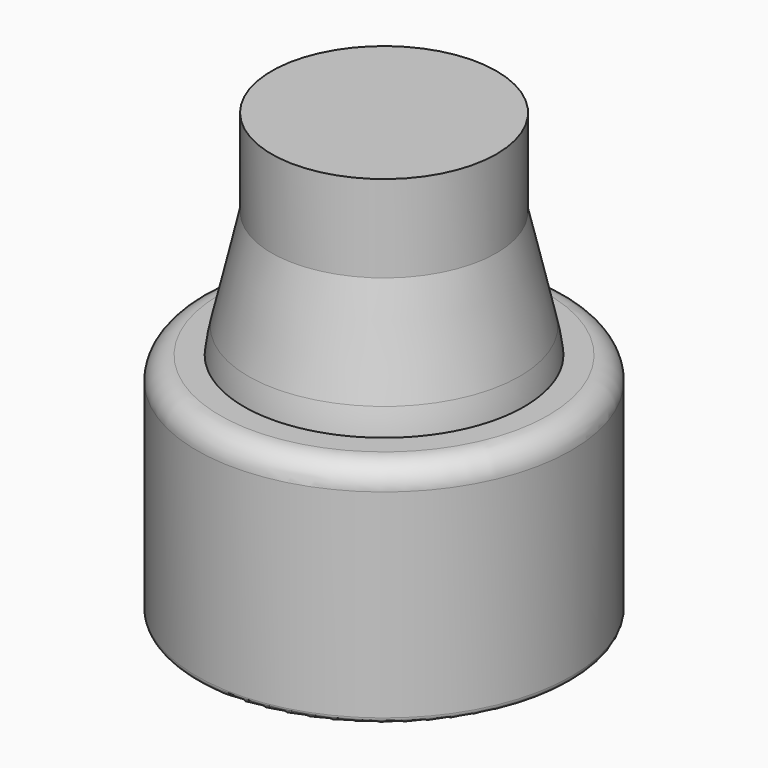
from build123d import *

# Parameters (mm, degrees)
F2_R     = 4.2825511293
F3_DEPTH = 7.85
F4_R     = 4
F5_DEPTH = 1
F5_TAPER = 70


# Not quite as in the source:
# - an extrude ends at something that could not be found from the text; its depth is read off the source's solid


with BuildPart() as f1:
    # F0 (on Front) → F1 (revolve)
    with BuildSketch(Plane.XZ):
        with BuildLine():
            Line((5.65, 7.85), (4, 7.85))
            Line((4, 7.85), (4, 4.75))
            Line((4, 4.75), (1.25, 3.1622867597))
            Line((1.25, 3.1622867597), (0, 3.1622867597))
            Line((0, 3.1622867597), (0, 0))
            Line((0, 0), (6.25, 0))
            ThreePointArc((6.25, 0), (6.3914213562, 0.0585786438), (6.45, 0.2))
            Line((6.45, 0.2), (6.45, 7.05))
            ThreePointArc((6.45, 7.05), (6.2156854249, 7.6156854249), (5.65, 7.85))
        make_face()
    revolve(axis=Axis((0, 0, 1.5811433799), (0, 0, -1)))

    # F2 (on face) → F3 (join, through all)
    with BuildSketch(Plane.XY.offset(7.85)):
        Circle(F2_R)
        with BuildLine():
            ThreePointArc((-0.772740661, 3.4070552361), (0, 4), (0.772740661, 3.4070552361))
            Line((0.772740661, 3.4070552361), (0.7889794079, 3.3464514079))
            ThreePointArc((0.7889794079, 3.3464514079), (1.4412755647, 2.4963625057), (2.5036222278, 2.3565019142))
            Line((2.5036222278, 2.3565019142), (2.564226056, 2.372740661))
            ThreePointArc((2.564226056, 2.372740661), (3.4641016151, 2), (3.3369667171, 1.0343145751))
            Line((3.3369667171, 1.0343145751), (3.2926016357, 0.9899494937))
            ThreePointArc((3.2926016357, 0.9899494937), (2.8825511293, 0), (3.2926016357, -0.9899494937))
            Line((3.2926016357, -0.9899494937), (3.3369667171, -1.0343145751))
            ThreePointArc((3.3369667171, -1.0343145751), (3.4641016151, -2), (2.564226056, -2.372740661))
            Line((2.564226056, -2.372740661), (2.5036222278, -2.3565019142))
            ThreePointArc((2.5036222278, -2.3565019142), (1.4412755647, -2.4963625057), (0.7889794079, -3.3464514079))
            Line((0.7889794079, -3.3464514079), (0.772740661, -3.4070552361))
            ThreePointArc((0.772740661, -3.4070552361), (0, -4), (-0.772740661, -3.4070552361))
            Line((-0.772740661, -3.4070552361), (-0.7889794079, -3.3464514079))
            ThreePointArc((-0.7889794079, -3.3464514079), (-1.4412755647, -2.4963625057), (-2.5036222278, -2.3565019142))
            Line((-2.5036222278, -2.3565019142), (-2.564226056, -2.372740661))
            ThreePointArc((-2.564226056, -2.372740661), (-3.4641016151, -2), (-3.3369667171, -1.0343145751))
            Line((-3.3369667171, -1.0343145751), (-3.2926016357, -0.9899494937))
            ThreePointArc((-3.2926016357, -0.9899494937), (-2.8825511293, 0), (-3.2926016357, 0.9899494937))
            Line((-3.2926016357, 0.9899494937), (-3.3369667171, 1.0343145751))
            ThreePointArc((-3.3369667171, 1.0343145751), (-3.4641016151, 2), (-2.564226056, 2.372740661))
            Line((-2.564226056, 2.372740661), (-2.5036222278, 2.3565019142))
            ThreePointArc((-2.5036222278, 2.3565019142), (-1.4412755647, 2.4963625057), (-0.7889794079, 3.3464514079))
            Line((-0.7889794079, 3.3464514079), (-0.772740661, 3.4070552361))
        make_face(mode=Mode.SUBTRACT)
    extrude(amount=-F3_DEPTH)

    # F4 (on face) → F5 (cut)
    with BuildSketch(Plane.XY.offset(7.85)):
        Circle(F4_R)
    extrude(amount=-F5_DEPTH, taper=F5_TAPER, mode=Mode.SUBTRACT)


with BuildPart() as f7:
    # F6 (on Front) → F7 (revolve)
    with BuildSketch(Plane.XZ):
        with BuildLine():
            Line((3.875, 15.2), (0, 15.2))
            Line((0, 15.2), (0, 0))
            Line((0, 0), (3.495, 0))
            Line((3.495, 0), (4.6778236218, 5.1233719814))
            ThreePointArc((4.6778236218, 5.1233719814), (4.8828631035, 6.9229804161), (4.6778236218, 8.7225888509))
            Line((4.6778236218, 8.7225888509), (3.875, 12.2))
            Line((3.875, 12.2), (3.875, 15.2))
        make_face()
    revolve(axis=Axis((0, 0, 7.6), (0, 0, -1)))


with BuildPart() as f9:
    # F8 (on Front) → F9 (revolve)
    with BuildSketch(Plane.XZ):
        with BuildLine():
            Line((0, 7.0269373127), (0, 0))
            Line((0, 0), (5.3425146232, 0))
            ThreePointArc((5.3425146232, 0), (5.679504679, 0.1306252549), (5.840417087, 0.4542491907))
            Line((5.840417087, 0.4542491907), (6.2935137888, 5.3852650008))
            ThreePointArc((6.2935137888, 5.3852650008), (6.3100029903, 6.2569191501), (6.2, 7.1217614432))
            ThreePointArc((6.2, 7.1217614432), (6.0365510119, 7.4013445877), (5.7360583301, 7.522118983))
            Line((5.7360583301, 7.522118983), (4.25, 7.6))
            Line((4.25, 7.6), (1, 7.0269373127))
            Line((1, 7.0269373127), (0, 7.0269373127))
        make_face()
    revolve(axis=Axis((0, 0, 3.5134686563), (0, 0, 1)))


solid = Compound([f1.part, f7.part, f9.part])
